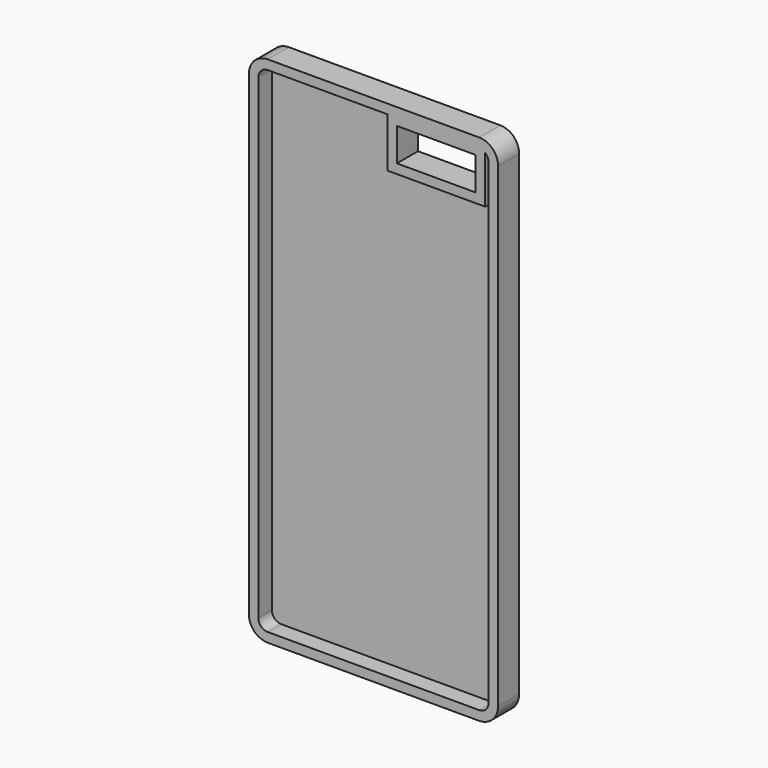
from build123d import *

# Parameters (mm, degrees)
F0_W        = 67.1
F0_H        = 138.3
F0_W_2      = 21.2295074016
F0_H_2      = 8.8934414089
F1_DEPTH    = 3.55
F2_R        = 5.08
F3_T        = 2.54
F3_T3_DEPTH = 12.18


# Not quite as in the source:
# - a shell that OpenCascade refuses in one call is made with other operations: the cavity is built on its own and cut out


with BuildPart() as f1:
    # F0 (on Front) → F1 (new body, symmetric)
    with BuildSketch(Plane.XZ):
        Rectangle(F0_W, F0_H)
        with Locations((16.9262299314, 60.2459032089)):
            Rectangle(F0_W_2, F0_H_2, mode=Mode.SUBTRACT)
    extrude(amount=F1_DEPTH, both=True)

    # F2
    f2_edges = [f1.edges().sort_by_distance(p)[0] for p in [
        (33.55, 0, 69.15),
        (-33.55, 0, 69.15),
        (33.55, 0, -69.15),
        (-33.55, 0, -69.15),
    ]]
    fillet(f2_edges, radius=F2_R)

    # F3: shell of thickness 2.54, made by hand


with BuildPart() as f3_core1:
    # F3_t2: copy of F1
    add(f1.part)

    # the walls: a layer under each face that stays
    f3_faces = [f3_core1.faces().sort_by_distance(p)[0] for p in [
        (0, 0, 69.15),
        (0, 3.55, 0),
        (32.0621024484, 0, 67.6621024484),
        (-32.0621024484, 0, 67.6621024484),
        (33.55, 0, 0),
        (-33.55, 0, 0),
        (32.0621024484, 0, -67.6621024484),
        (-32.0621024484, 0, -67.6621024484),
        (0, 0, -69.15),
        (6.3114762306, 0, 60.2459032089),
        (16.9262299314, 0, 64.6926239133),
        (27.5409836322, 0, 60.2459032089),
        (16.9262299314, 0, 55.7991825044),
    ]]
    thicken(f3_faces, amount=-F3_T, mode=Mode.SUBTRACT)

    # F3_s4 → F3_t3 (cut)
    with BuildSketch(Plane.XZ.offset(-6.09)):
        Polygon((6.3368762306, 64.6672239133), (3.7714762306, 64.6926239133), (3.7714762306, 67.2326239133), (6.3114762306, 67.2326239133), align=None)
        Polygon((6.3368762306, 55.8245825044), (3.7714762306, 55.7991825044), (3.7714762306, 53.2591825044), (6.3114762306, 53.2591825044), align=None)
        Polygon((27.5155836322, 64.6672239133), (27.5409836322, 67.2326239133), (30.0809836322, 67.2326239133), (30.0809836322, 64.6926239133), align=None)
        Polygon((27.5155836322, 55.8245825044), (30.0809836322, 55.7991825044), (30.0809836322, 53.2591825044), (27.5409836322, 53.2591825044), align=None)
    extrude(amount=F3_T3_DEPTH, mode=Mode.SUBTRACT)


with BuildPart() as f1_1:
    add(f1.part)

    # what is left inside the walls is the cavity
    f3_cavity = [f3_core1.part.solids().sort_by_distance(p)[0] for p in [
        (0, -3.5246, -22.203333),
    ]]
    add(f3_cavity, mode=Mode.SUBTRACT)


solid = f1_1.part
